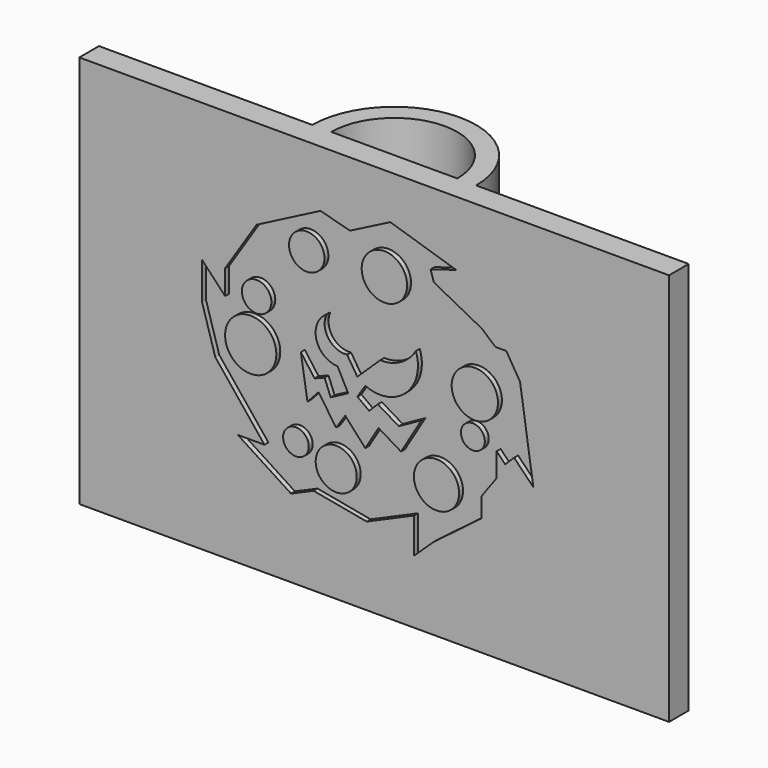
from build123d import *

# Parameters (mm, degrees)
F0_W     = 76.2
F0_H     = 50.8
F1_DEPTH = 3.175
F2_R     = 1.6558767695
F2_R_2   = 2.6518381977
F2_R_3   = 3.3103533059
F2_R_4   = 2.921000123
F2_R_5   = 1.5450229593
F2_R_6   = 1.9050003029
F2_R_7   = 2.2895237278
F2_R_8   = 2.9892250919
F2_R_9   = 2.9320238784
F3_DEPTH = 0.635
F5_DEPTH = 50.8


# Not quite as in the source:
# - a feature names something its author has since deleted; it is built from what else it names


with BuildPart() as f1:
    # F0 (on Front) → F1 (new body)
    with BuildSketch(Plane.XZ):
        with Locations((38.1, 25.4)):
            Rectangle(F0_W, F0_H)
    extrude(amount=F1_DEPTH)

    # F2 (on face) → F3 (cut)
    with BuildSketch(Plane.XZ.offset(3.175)):
        Polygon((48.691868487, 42.4682941364), (40.1828733117, 45.1352943044), (34.9758711487, 42.4682941364), (31.1658705429, 43.4842941893), (22.9070743114, 39.2204960176), (18.8385191247, 32.9432937858), (18.8385191247, 29.7757912988), (15.8623714775, 32.9432937858), (15.8623714775, 28.1172938255), (17.5768719597, 22.418530716), (23.9268724651, 14.5282934961), (20.4978712678, 14.5282934961), (27.3558708683, 10.0832957385), (30.27687006, 11.35329563), (37.1348724544, 10.0832957385), (43.2308704436, 12.7502943931), (43.2308704436, 8.1782940386), (45.7990180271, 10.59129495), (51.9938726753, 15.2902941761), (51.9938726753, 17.8302939592), (53.930624873, 20.4972944764), (53.930624873, 23.545293471), (55.0292181151, 22.418530716), (56.1848726899, 23.545293471), (58.6613714775, 21.005293688), (56.9468696446, 32.435293643), (55.1688742668, 35.356293766), (53.7718717784, 35.356293766), (51.9938726753, 36.8802941946), (45.7990180271, 40.1225700636), (45.3898717493, 41.4522940835), align=None)
        with Locations((27.9908708141, 16.1792937277)):
            Circle(F2_R, mode=Mode.SUBTRACT)
        with Locations((33.1978739083, 14.7822949646)):
            Circle(F2_R_2, mode=Mode.SUBTRACT)
        with Locations((22.1488724307, 25.3232944367)):
            Circle(F2_R_3, mode=Mode.SUBTRACT)
        with BuildLine():
            Line((29.4827647798, 21.2285935147), (28.6258707598, 26.5932943282))
            Line((28.6258707598, 26.5932943282), (30.4038726569, 24.1802934168))
            Line((30.4038726569, 24.1802934168), (31.6916008863, 24.6882943394))
            Line((31.6916008863, 24.6882943394), (32.4751487195, 22.7020840415))
            Line((32.4751487195, 22.7020840415), (34.7450423849, 23.8972995039))
            Line((34.7450423849, 23.8972995039), (33.3584630646, 26.5306218754))
            ThreePointArc((33.3584630646, 26.5306218754), (30.6271191315, 28.6945286164), (31.9278740168, 31.9272935001))
            ThreePointArc((31.9278740168, 31.9272935001), (32.188274126, 29.3087235679), (34.5948708088, 28.2442945597))
            Line((34.5948708088, 28.2442945597), (35.9297474949, 26.173913466))
            Line((35.9297474949, 26.173913466), (38.8855502865, 29.0062933771))
            ThreePointArc((38.8855502865, 29.0062933771), (41.5322516722, 29.6478879221), (43.484871912, 31.5462940914))
            ThreePointArc((43.484871912, 31.5462940914), (42.2018854798, 26.3705417725), (36.9460296513, 25.4702941614))
            Line((36.9460296513, 25.4702941614), (35.9297474949, 23.8972995039))
            Line((35.9297474949, 23.8972995039), (37.4565196476, 22.7832946537))
            Line((37.4565196476, 22.7832946537), (38.571963384, 23.8972995039))
            Line((38.571963384, 23.8972995039), (41.2807169848, 22.2783325716))
            Line((41.2807169848, 22.2783325716), (44.2106343052, 23.8972995039))
            Line((44.2106343052, 23.8972995039), (41.5642807871, 19.4857340033))
            Line((41.5642807871, 19.4857340033), (38.6588719517, 21.2285935147))
            Line((38.6588719517, 21.2285935147), (36.9460296513, 18.3732244384))
            Line((36.9460296513, 18.3732244384), (34.3611069299, 21.2285935147))
            Line((34.3611069299, 21.2285935147), (33.1806698754, 19.4857340033))
            Line((33.1806698754, 19.4857340033), (30.9118700058, 22.7832946537))
            Line((30.9118700058, 22.7832946537), (29.4827647798, 21.2285935147))
        make_face(mode=Mode.SUBTRACT)
        with Locations((46.1518705666, 17.1952940134)):
            Circle(F2_R_4, mode=Mode.SUBTRACT)
        with Locations((50.8508716554, 24.1802934168)):
            Circle(F2_R_5, mode=Mode.SUBTRACT)
        with Locations((22.9108707823, 31.0382939485)):
            Circle(F2_R_6, mode=Mode.SUBTRACT)
        with Locations((29.3878714398, 38.277293889)):
            Circle(F2_R_7, mode=Mode.SUBTRACT)
        with Locations((51.1048731238, 29.1332941113)):
            Circle(F2_R_8, mode=Mode.SUBTRACT)
        with Locations((39.4208707691, 38.658294229)):
            Circle(F2_R_9, mode=Mode.SUBTRACT)
    extrude(amount=-F3_DEPTH, mode=Mode.SUBTRACT)

    # F4 (on Top) → F5 (join)
    with BuildSketch(Plane.XY):
        with BuildLine():
            ThreePointArc((30.0156539358, 0), (38.1572704301, 8.1416164943), (46.2988869244, 0))
            Line((46.2988869244, 0), (48.7363704301, 0))
            ThreePointArc((48.7363704301, 0), (38.1572704301, 10.5791), (27.5781704301, 0))
            Line((27.5781704301, 0), (30.0156539358, 0))
        make_face()
    extrude(amount=F5_DEPTH)


solid = f1.part
